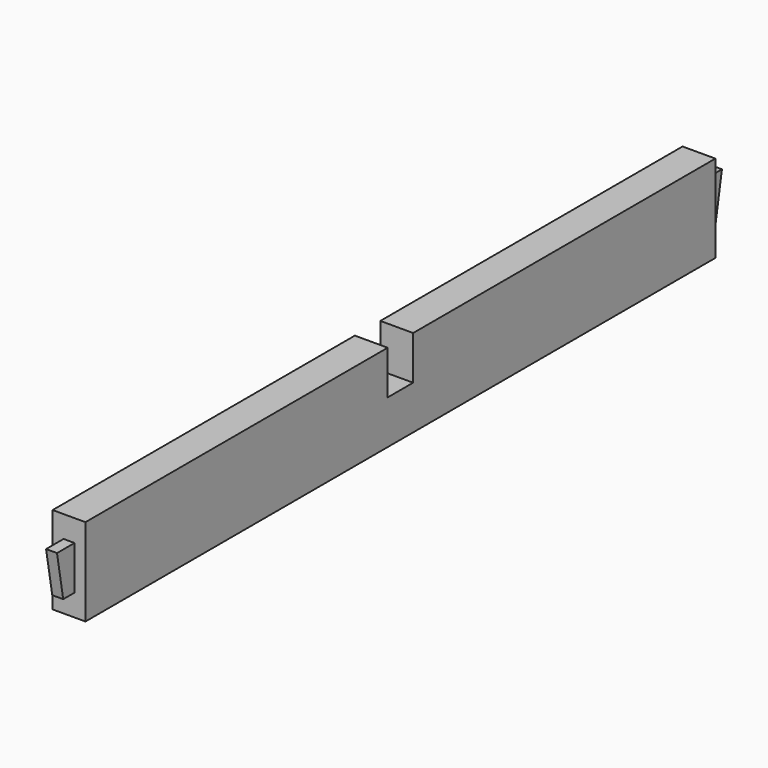
from build123d import *

# Parameters (mm, degrees)
F0_W     = 457.2
F0_H     = 50.8
F1_DEPTH = 9.525
F2_W     = 19.05
F2_H     = 18.4890627861
F3_DEPTH = 25.4
F4_W     = 6.35
F4_H     = 25.4
F5_DEPTH = 12.7
F6_W     = 6.35
F6_H     = 25.4
F7_DEPTH = 12.7
F8_SIZE2 = 4.478695
F8_SIZE  = 25.39999
F9_SIZE2 = 4.478695
F9_SIZE  = 25.39999


# Not quite as in the source:
# - a fillet or chamfer is up to 0.001 mm smaller than in the source, because OpenCascade refuses the exact size


with BuildPart() as f1:
    # F0 (on Right) → F1 (new body, symmetric)
    with BuildSketch(Plane.YZ):
        Rectangle(F0_W, F0_H)
    extrude(amount=F1_DEPTH, both=True)

    # F2 (on face) → F3 (cut, symmetric)
    with BuildSketch(Plane.XY.offset(25.4)):
        Rectangle(F2_W, F2_H)
    extrude(amount=F3_DEPTH, both=True, mode=Mode.SUBTRACT)

    # F4 (on face) → F5 (join, symmetric)
    with BuildSketch(Plane.XZ.offset(228.6)):
        Rectangle(F4_W, F4_H)
    extrude(amount=F5_DEPTH, both=True)

    # F6 (on face) → F7 (join, symmetric)
    with BuildSketch(Plane(origin=(0, 228.6, 0), x_dir=(-1, 0, 0), z_dir=(0, 1, 0))):
        Rectangle(F6_W, F6_H)
    extrude(amount=F7_DEPTH, both=True)

    # F8 (size 25.4 and 4.47870531 in the source; OpenCascade refuses exactly that, so slightly less here)
    f8_edges = [f1.edges().sort_by_distance(p)[0] for p in [
        (0, 241.3, -12.7),
    ]]
    f8_side = f1.faces().sort_by_distance((0, 241.3, 0))[0]
    chamfer(f8_edges, length=F8_SIZE, length2=F8_SIZE2, reference=f8_side)

    # F9 (size 25.4 and 4.47870531 in the source; OpenCascade refuses exactly that, so slightly less here)
    f9_edges = [f1.edges().sort_by_distance(p)[0] for p in [
        (0, -241.3, -12.7),
    ]]
    f9_side = f1.faces().sort_by_distance((0, -241.3, 0))[0]
    chamfer(f9_edges, length=F9_SIZE, length2=F9_SIZE2, reference=f9_side)


solid = f1.part
